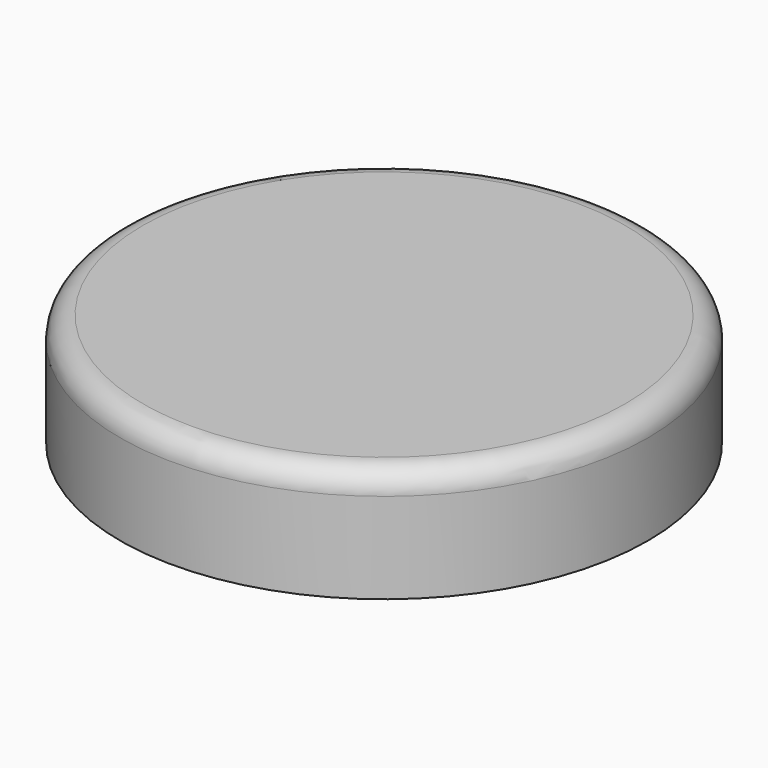
from build123d import *

# Parameters (mm, degrees)
F0_R     = 59.2365413748
F1_DEPTH = 25.4
F2_R     = 5.08


# Not quite as in the source:
# - a feature names something its author has since deleted; it is built from what else it names


with BuildPart() as f1:
    # F0 (on Top) → F1 (new body)
    with BuildSketch(Plane.XY):
        with Locations((-124.2445409298, 9.3189002946)):
            Circle(F0_R)
    extrude(amount=F1_DEPTH)

    # F2
    f2_edges = [f1.edges().sort_by_distance(p)[0] for p in [
        (-183.481082, 9.3189, 25.4),
    ]]
    fillet(f2_edges, radius=F2_R)


solid = f1.part
